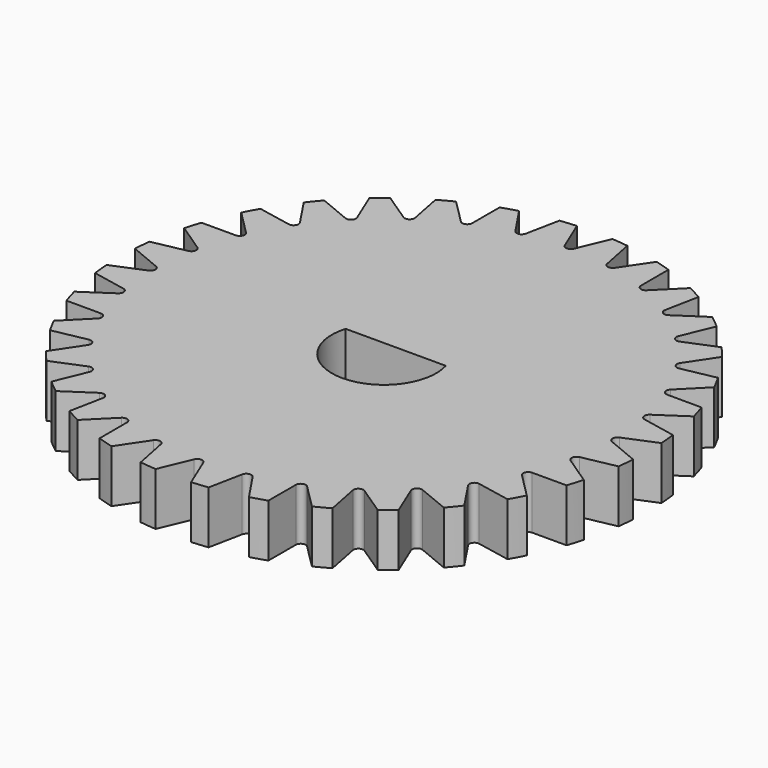
from build123d import *

# Parameters (mm, degrees)
F0_R            = 15.8688012495
F1_DEPTH        = 3.175
F3_DEPTH        = 3.175
F3_COPIES_COUNT = 32


# Not quite as in the source:
# - a pattern or mirror of a feature is missing from the dataset's text; its kind, count and spacing are read off the source's solid


with BuildPart() as f1:
    # F0 (on Top) → F1 (new body)
    with BuildSketch(Plane.XY):
        Circle(F0_R)
        with BuildLine():
            ThreePointArc((3.0120159229, 0.8763), (0, -3.1369), (-3.0120159229, 0.8763))
            Line((-3.0120159229, 0.8763), (3.0120159229, 0.8763))
        make_face(mode=Mode.SUBTRACT)
    extrude(amount=F1_DEPTH)

    # F2 (on face) → F3 (cut, through all)
    with BuildSketch(Plane.XY.offset(3.175)):
        with BuildLine():
            Line((-13.9312413972, 0.274735453), (-15.8329891451, 1.065508248))
            ThreePointArc((-15.8329891451, 1.065508248), (-15.8688012495, 0), (-15.8329891451, -1.065508248))
            Line((-15.8329891451, -1.065508248), (-13.9312413972, -0.274735453))
            ThreePointArc((-13.9312413972, -0.274735453), (-13.747940143, 0), (-13.9312413972, 0.274735453))
        make_face()
    f3 = extrude(amount=-F3_DEPTH, mode=Mode.SUBTRACT)

    # F3_copies: F3 ×32 about axis
    f3_copies_axis = Axis((0, 0, 0), (0, 0, 1))
    for i in range(1, F3_COPIES_COUNT):
        add(f3.rotate(f3_copies_axis, i * 360 / F3_COPIES_COUNT), mode=Mode.SUBTRACT)


solid = f1.part
